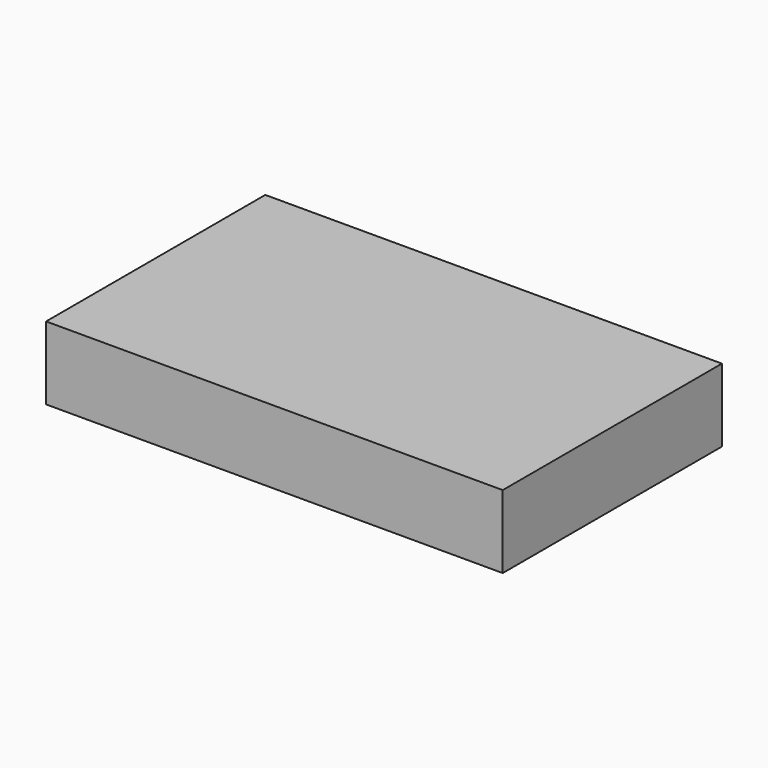
from build123d import *

# Parameters (mm, degrees)
F0_W     = 250
F0_H     = 40
F1_DEPTH = 150
F2_T     = -2.5


# Not quite as in the source:
# - the program builds the solid bodies; features that only make, move or delete a surface that nothing else refers to are left out


with BuildPart() as f1:
    # F0 (on Front) → F1 (new body)
    with BuildSketch(Plane.XZ):
        with Locations((-125, 20)):
            Rectangle(F0_W, F0_H)
    extrude(amount=-F1_DEPTH)

    # F2
    f2_openings = [f1.faces().sort_by_distance(p)[0] for p in [
        (-125, 75, 0),
    ]]
    offset(amount=F2_T, openings=f2_openings)


solid = f1.part
